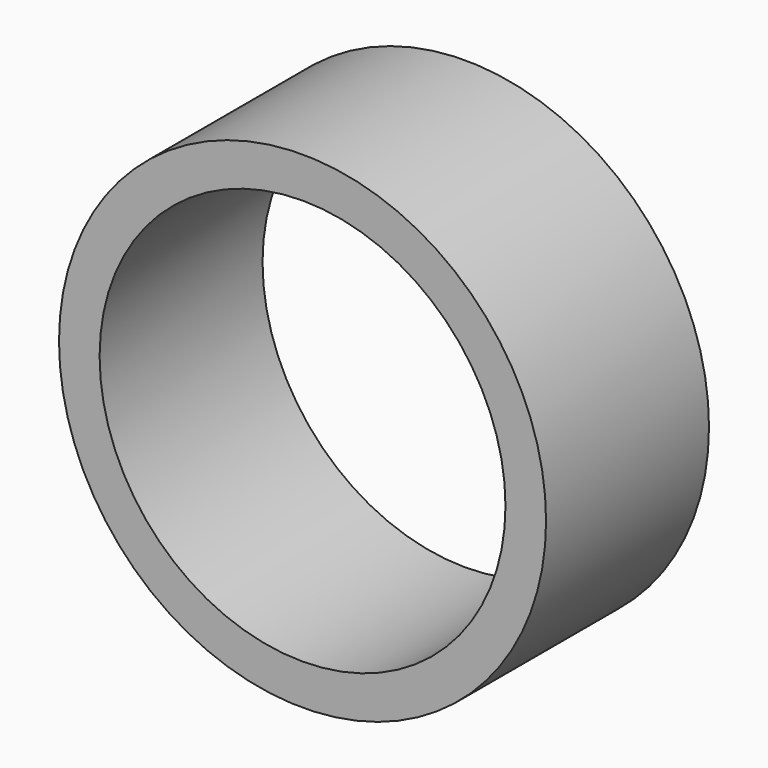
from build123d import *

# Parameters (mm, degrees)
F0_R     = 72.2228243582
F1_DEPTH = 10
F2_R     = 72.2228243582
F3_DEPTH = 25.4
F5_R     = 13.3709609509
F6_DEPTH = 226
F4_R     = 60.1818073618
F7_DEPTH = 139.5800691098
F8_DEPTH = 25


# Not quite as in the source:
# - an extrude ends at something that could not be found from the text; its depth is read off the source's solid


with BuildPart() as f1:
    # F0 (on Front) → F1 (new body)
    with BuildSketch(Plane.XZ):
        Circle(F0_R)
    extrude(amount=F1_DEPTH)

    # F2 (on face) → F3 (join)
    with BuildSketch(Plane.XZ.offset(10)):
        Circle(F2_R)
    extrude(amount=F3_DEPTH)

    # F5 (on Front) → F6 (cut, through all)
    with BuildSketch(Plane.XZ):
        with Locations((0, 13.3709609509)):
            Circle(F5_R)
    extrude(amount=-F6_DEPTH, mode=Mode.SUBTRACT)

    # F4 (on face) → F7 (cut)
    with BuildSketch(Plane(origin=(0, 0, 0), x_dir=(-1, 0, 0), z_dir=(0, 1, 0))):
        Circle(F4_R)
    extrude(amount=-F7_DEPTH, mode=Mode.SUBTRACT)

    # F8 (add): a face of the model
    f8_faces = [f1.faces().sort_by_distance(p)[0] for p in [
        (-70.1800544038, -35.4, 0),
    ]]
    extrude(f8_faces, amount=F8_DEPTH)


solid = f1.part
